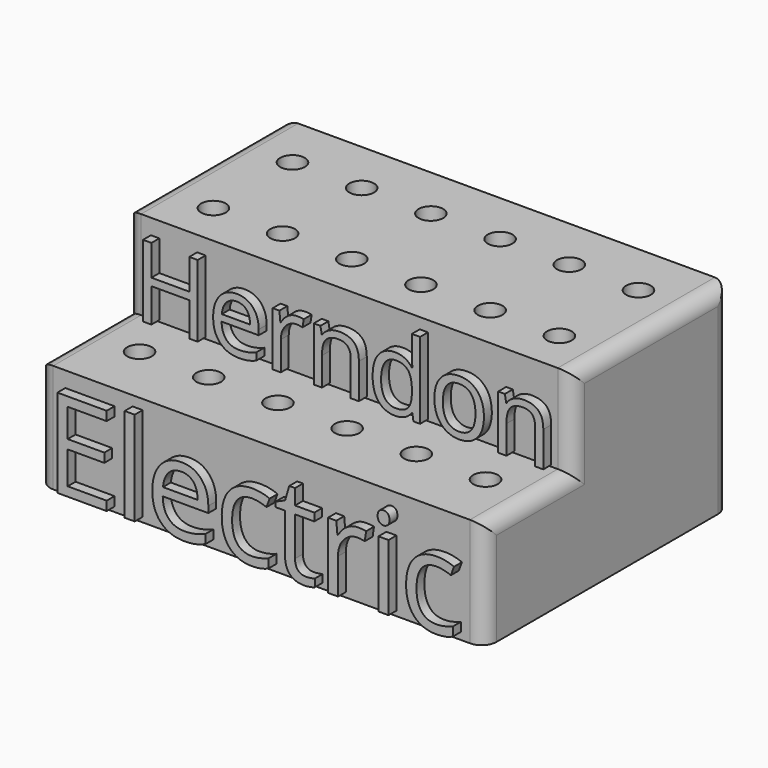
from build123d import *

# Parameters (mm, degrees)
F0_W         = 114.6860048175
F0_H         = 50.4378248006
F1_DEPTH     = 50.8
F0_H_2       = 28.2211601734
F2_DEPTH     = 27.94
F3_D         = 6.35
F4_T         = -2.54
F5_T1_DEPTH  = 37.7461601734
F5_T3_DEPTH  = 69.4878248006
F5_T5_DEPTH  = 32.385
F5_T7_DEPTH  = 46.99
F5_T9_DEPTH  = 69.85
F5_T15_DEPTH = 41.91
F5_T19_DEPTH = 47.2711601734
F5_T26_DEPTH = 41.91
F5_T30_DEPTH = 47.2711601734
F6_TEXT_SIZE = 25.8867559816
F7_TEXT_SIZE = 31.7880140486
F8_DEPTH     = 2.54


# Not quite as in the source:
# - a fillet or chamfer that OpenCascade refuses, or shapes differently, is made with other operations: its cross-section is extruded or revolved along the edge and cut away or added
# - Text() gives the source's letters only with a copy of the font that has no kerning and outlines rounded to 1/6400 em; it was checked with that copy


with BuildPart() as f1:
    # F0 (on Top) → F1 (new body)
    with BuildSketch(Plane.XY):
        with Locations((12.6094557345, 3.7528136745)):
            Rectangle(F0_W, F0_H)
    extrude(amount=F1_DEPTH)

    # F0 (on Top) → F2 (join)
    with BuildSketch(Plane.XY):
        with Locations((12.6094557345, -35.5766788125)):
            Rectangle(F0_W, F0_H_2)
    extrude(amount=F2_DEPTH)

    # F3 (through all)
    with Locations(Plane(origin=(0, 0, 0), x_dir=(1, 0, 0), z_dir=(0, 0, -1))):
        with Locations((-31.2234144658, -15.0422326565), (-13.4434144658, -15.0422326565), (4.3365855342, -15.0422326565), (22.1165855342, -15.0422326565), (39.8965855342, -15.0422326565), (57.6765855342, -15.0422326565), (57.6765855342, 10.3577673435), (57.6765855342, 34.0755544603), (39.8965855342, 34.0755544603), (22.1165855342, 34.0755544603), (4.3365855342, 34.0755544603), (-13.4434144658, 34.0755544603), (-31.2234144658, 34.0755544603), (-31.2234144658, 10.3577673435), (-13.4434144658, 10.3577673435), (4.3365855342, 10.3577673435), (22.1165855342, 10.3577673435), (39.8965855342, 10.3577673435)):
            Hole(F3_D / 2)

    # F4
    f4_openings = [f1.faces().sort_by_distance(p)[0] for p in [
        (12.609456, 28.971726, 25.4),
    ]]
    offset(amount=F4_T, openings=f4_openings, kind=Kind.INTERSECTION)

    # F5: fillet of radius 3.81 on 10 edges, made by hand

    # F5_s2 → F5_t1 (cut)
    with BuildSketch(Plane.XZ.offset(21.4660987258)):
        with BuildLine():
            ThreePointArc((69.9524581432, 24.13), (68.8365349796, 26.8240768363), (66.1424581432, 27.94))
            Line((66.1424581432, 27.94), (69.9524581432, 27.94))
            Line((69.9524581432, 27.94), (69.9524581432, 24.13))
        make_face()
        with BuildLine():
            ThreePointArc((-44.7335466743, 24.13), (-43.6176235106, 26.8240768363), (-40.9235466743, 27.94))
            Line((-40.9235466743, 27.94), (-44.7335466743, 27.94))
            Line((-44.7335466743, 27.94), (-44.7335466743, 24.13))
        make_face()
    extrude(amount=F5_T1_DEPTH, mode=Mode.SUBTRACT)

    # F5_s4 → F5_t3 (cut)
    with BuildSketch(Plane.XZ.offset(-38.4967260748)):
        with BuildLine():
            ThreePointArc((69.9524581432, 46.99), (68.8365349796, 49.6840768363), (66.1424581432, 50.8))
            Line((66.1424581432, 50.8), (69.9524581432, 50.8))
            Line((69.9524581432, 50.8), (69.9524581432, 46.99))
        make_face()
        with BuildLine():
            ThreePointArc((-44.7335466743, 46.99), (-43.6176235106, 49.6840768363), (-40.9235466743, 50.8))
            Line((-40.9235466743, 50.8), (-44.7335466743, 50.8))
            Line((-44.7335466743, 50.8), (-44.7335466743, 46.99))
        make_face()
    extrude(amount=F5_T3_DEPTH, mode=Mode.SUBTRACT)

    # F5_s6 → F5_t5 (cut)
    with BuildSketch(Plane.XY.offset(27.94)):
        with BuildLine():
            ThreePointArc((69.9524581432, -17.6560987258), (68.8365349796, -20.3501755621), (66.1424581432, -21.4660987258))
            Line((66.1424581432, -21.4660987258), (69.9524581432, -21.4660987258))
            Line((69.9524581432, -21.4660987258), (69.9524581432, -17.6560987258))
        make_face()
        with BuildLine():
            ThreePointArc((-44.7335466743, -17.6560987258), (-43.6176235106, -20.3501755621), (-40.9235466743, -21.4660987258))
            Line((-40.9235466743, -21.4660987258), (-44.7335466743, -21.4660987258))
            Line((-44.7335466743, -21.4660987258), (-44.7335466743, -17.6560987258))
        make_face()
    extrude(amount=F5_T5_DEPTH, mode=Mode.SUBTRACT)

    # F5_s8 → F5_t7 (cut)
    with BuildSketch(Plane.XY.offset(-9.525)):
        with BuildLine():
            ThreePointArc((69.9524581432, -45.8772588992), (68.8365349796, -48.5713357355), (66.1424581432, -49.6872588992))
            Line((66.1424581432, -49.6872588992), (69.9524581432, -49.6872588992))
            Line((69.9524581432, -49.6872588992), (69.9524581432, -45.8772588992))
        make_face()
        with BuildLine():
            ThreePointArc((-44.7335466743, -45.8772588992), (-43.6176235106, -48.5713357355), (-40.9235466743, -49.6872588992))
            Line((-40.9235466743, -49.6872588992), (-44.7335466743, -49.6872588992))
            Line((-44.7335466743, -49.6872588992), (-44.7335466743, -45.8772588992))
        make_face()
    extrude(amount=F5_T7_DEPTH, mode=Mode.SUBTRACT)

    # F5_s10 → F5_t9 (cut)
    with BuildSketch(Plane.XY.offset(-9.525)):
        with BuildLine():
            ThreePointArc((69.9524581432, 25.1617260748), (68.8365349796, 27.8558029111), (66.1424581432, 28.9717260748))
            Line((66.1424581432, 28.9717260748), (69.9524581432, 28.9717260748))
            Line((69.9524581432, 28.9717260748), (69.9524581432, 25.1617260748))
        make_face()
        with BuildLine():
            ThreePointArc((-44.7335466743, 25.1617260748), (-43.6176235106, 27.8558029111), (-40.9235466743, 28.9717260748))
            Line((-40.9235466743, 28.9717260748), (-44.7335466743, 28.9717260748))
            Line((-44.7335466743, 28.9717260748), (-44.7335466743, 25.1617260748))
        make_face()
    extrude(amount=F5_T9_DEPTH, mode=Mode.SUBTRACT)


with BuildPart() as f5_tool13:
    # F5_s14 → F5_t15 (new body)
    with BuildSketch(Plane.XY.offset(18.415)):
        with BuildLine():
            ThreePointArc((69.9524581432, -17.6560987258), (68.8365349796, -20.3501755621), (66.1424581432, -21.4660987258))
            Line((66.1424581432, -21.4660987258), (69.9524581432, -21.4660987258))
            Line((69.9524581432, -21.4660987258), (69.9524581432, -17.6560987258))
        make_face()
    extrude(amount=F5_T15_DEPTH)

    split(bisect_by=Plane.XY.offset(27.94), keep=Keep.BOTTOM)


with BuildPart() as f5_tool17:
    # F5_s18 → F5_t19 (new body)
    with BuildSketch(Plane.XZ.offset(59.2122588992)):
        with BuildLine():
            ThreePointArc((69.9524581432, 24.13), (68.8365349796, 26.8240768363), (66.1424581432, 27.94))
            Line((66.1424581432, 27.94), (69.9524581432, 27.94))
            Line((69.9524581432, 27.94), (69.9524581432, 24.13))
        make_face()
    extrude(amount=-F5_T19_DEPTH)

    split(bisect_by=Plane.XZ.offset(21.4660987258), keep=Keep.BOTTOM)


with BuildPart() as f5_tool13_1:
    add(f5_tool13.part)

    # F5_t21: intersect F5_tool17
    add(f5_tool17.part, mode=Mode.INTERSECT)


with BuildPart() as f1_1:
    add(f1.part)

    # F5_t11: cut F5_tool13
    add(f5_tool13_1.part, mode=Mode.SUBTRACT)


with BuildPart() as f5_tool24:
    # F5_s25 → F5_t26 (new body)
    with BuildSketch(Plane.XY.offset(18.415)):
        with BuildLine():
            ThreePointArc((-44.7335466743, -17.6560987258), (-43.6176235106, -20.3501755621), (-40.9235466743, -21.4660987258))
            Line((-40.9235466743, -21.4660987258), (-44.7335466743, -21.4660987258))
            Line((-44.7335466743, -21.4660987258), (-44.7335466743, -17.6560987258))
        make_face()
    extrude(amount=F5_T26_DEPTH)

    split(bisect_by=Plane.XY.offset(27.94), keep=Keep.BOTTOM)


with BuildPart() as f5_tool28:
    # F5_s29 → F5_t30 (new body)
    with BuildSketch(Plane.XZ.offset(11.9410987258)):
        with BuildLine():
            ThreePointArc((-44.7335466743, 24.13), (-43.6176235106, 26.8240768363), (-40.9235466743, 27.94))
            Line((-40.9235466743, 27.94), (-44.7335466743, 27.94))
            Line((-44.7335466743, 27.94), (-44.7335466743, 24.13))
        make_face()
    extrude(amount=F5_T30_DEPTH)

    split(bisect_by=Plane.XZ.offset(21.4660987258), keep=Keep.BOTTOM)


with BuildPart() as f5_tool24_1:
    add(f5_tool24.part)

    # F5_t32: intersect F5_tool28
    add(f5_tool28.part, mode=Mode.INTERSECT)


with BuildPart() as f1_2:
    add(f1_1.part)

    # F5_t22: cut F5_tool24
    add(f5_tool24_1.part, mode=Mode.SUBTRACT)

    # F6 (on face) + F7 (on face) → F8 (join)
    with BuildSketch(Plane.XZ.offset(21.4660987258)):
        with Locations((-40.9235466743, 28.3515356933)):
            Text('Herndon', F6_TEXT_SIZE, font='Open Sans', text_align=(TextAlign.LEFT, TextAlign.BOTTOM))
    with BuildSketch(Plane.XZ.offset(49.6872588992)):
        with Locations((-40.9235466743, 1.242629885)):
            Text('Electric', F7_TEXT_SIZE, font='Open Sans', text_align=(TextAlign.LEFT, TextAlign.BOTTOM))
    extrude(amount=F8_DEPTH)


solid = f1_2.part
